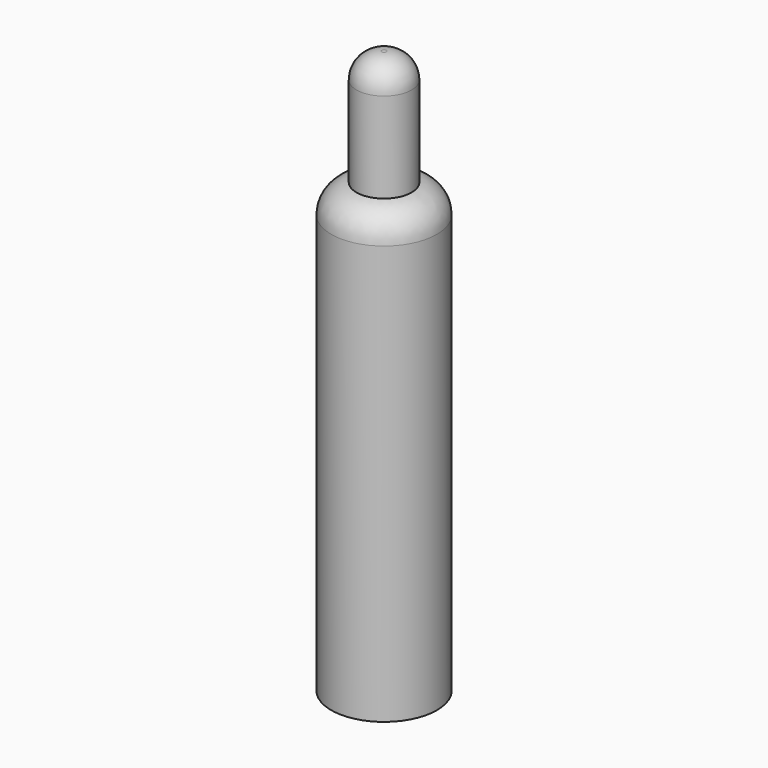
from build123d import *

# Parameters (mm, degrees)
F0_R     = 92.9783177543
F1_DEPTH = 787.4
F2_R     = 48.5104266544
F3_DEPTH = 203.2
F4_R     = 44.45


# Not quite as in the source:
# - a fillet or chamfer that OpenCascade refuses, or shapes differently, is made with other operations: its cross-section is extruded or revolved along the edge and cut away or added


with BuildPart() as f1:
    # F0 (on Top) → F1 (new body)
    with BuildSketch(Plane.XY):
        Circle(F0_R)
    extrude(amount=F1_DEPTH)

    # F2 (on face) → F3 (join)
    with BuildSketch(Plane.XY.offset(787.4)):
        Circle(F2_R)
    extrude(amount=F3_DEPTH)

    # F4
    f4_edges = [f1.edges().sort_by_distance(p)[0] for p in [
        (-48.510427, 0, 990.6),
    ]]
    fillet(f4_edges, radius=F4_R)

    # F5: fillet of radius 50.8 on 1 edges, made by hand

    # F5_s1 → F5_t2 (revolve, cut)
    with BuildSketch(Plane.XZ):
        with BuildLine():
            ThreePointArc((48.5104266544, 787.4), (80.2723535875, 770.6039898535), (92.9783177543, 736.9961866832))
            Line((92.9783177543, 736.9961866832), (92.9783177543, 787.4))
            Line((92.9783177543, 787.4), (48.5104266544, 787.4))
        make_face()
    revolve(axis=Axis((0, 0, 787.4), (0, 0, 1)), mode=Mode.SUBTRACT)


solid = f1.part
